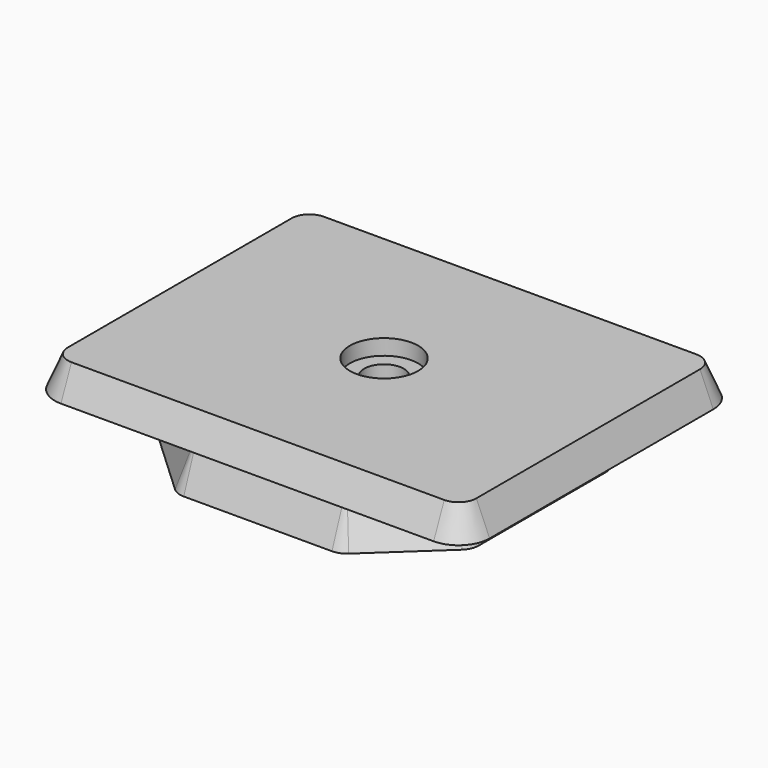
from build123d import *

# Parameters (mm, degrees)
F1_DEPTH       = 8.15
F1_TAPER       = 20
F2_T           = -4
F4_DEPTH       = 5
F4_TAPER       = 23
F6_D           = 6.35
F6_CBORE_D     = 11
F6_CBORE_DEPTH = 2.5


with BuildPart() as f1:
    # F0 (on Top) → F1 (new body)
    with BuildSketch(Plane.XY):
        with BuildLine():
            ThreePointArc((13.5235004185, 24.6379186874), (12.605417789, 25.1846935831), (11.5539321881, 25.375))
            Line((11.5539321881, 25.375), (-12.9567069347, 25.375))
            ThreePointArc((-12.9567069347, 25.375), (-14.1999477217, 25.1052659844), (-15.2196256222, 24.3445682304))
            Line((-15.2196256222, 24.3445682304), (-24.6379186874, 13.5235004185))
            ThreePointArc((-24.6379186874, 13.5235004185), (-25.1846935831, 12.605417789), (-25.375, 11.5539321881))
            Line((-25.375, 11.5539321881), (-25.375, -12.6529412227))
            ThreePointArc((-25.375, -12.6529412227), (-25.1255957189, -13.8505318001), (-24.4188512059, -14.8489995662))
            Line((-24.4188512059, -14.8489995662), (-13.972783394, -24.5710583435))
            ThreePointArc((-13.972783394, -24.5710583435), (-13.0270726549, -25.1667893035), (-11.9289321881, -25.375))
            Line((-11.9289321881, -25.375), (11.9289321881, -25.375))
            ThreePointArc((11.9289321881, -25.375), (13.0270726549, -25.1667893035), (13.972783394, -24.5710583435))
            Line((13.972783394, -24.5710583435), (24.4188512059, -14.8489995662))
            ThreePointArc((24.4188512059, -14.8489995662), (25.1255957189, -13.8505318001), (25.375, -12.6529412227))
            Line((25.375, -12.6529412227), (25.375, 12.9567069347))
            ThreePointArc((25.375, 12.9567069347), (25.1052659844, 14.1999477217), (24.3445682304, 15.2196256222))
            Line((24.3445682304, 15.2196256222), (13.5235004185, 24.6379186874))
        make_face()
    extrude(amount=F1_DEPTH, taper=F1_TAPER)

    # F2
    f2_openings = [f1.faces().sort_by_distance(p)[0] for p in [
        (0.016382, 0.006023, 0),
    ]]
    offset(amount=F2_T, openings=f2_openings)

    # F3 (on face) → F4 (join)
    with BuildSketch(Plane.XY.offset(8.15)):
        with BuildLine():
            ThreePointArc((35, 22.5), (33.5355339059, 26.0355339059), (30, 27.5))
            Line((30, 27.5), (-30, 27.5))
            ThreePointArc((-30, 27.5), (-33.5355339059, 26.0355339059), (-35, 22.5))
            Line((-35, 22.5), (-35, -22.5))
            ThreePointArc((-35, -22.5), (-33.5355339059, -26.0355339059), (-30, -27.5))
            Line((-30, -27.5), (30, -27.5))
            ThreePointArc((30, -27.5), (33.5355339059, -26.0355339059), (35, -22.5))
            Line((35, -22.5), (35, 22.5))
        make_face()
        with BuildLine():
            Line((11.5760193141, 22.4003768158), (22.397087126, 12.9820837505))
            ThreePointArc((22.397087126, 12.9820837505), (22.4056177404, 12.9706488817), (22.4086425907, 12.9567069347))
            Line((22.4086425907, 12.9567069347), (22.4086425907, -12.6529412227))
            ThreePointArc((22.4086425907, -12.6529412227), (22.405845722, -12.6663712392), (22.3979201499, -12.6775682533))
            Line((22.3979201499, -12.6775682533), (11.951852338, -22.3996270307))
            ThreePointArc((11.951852338, -22.3996270307), (11.9412469516, -22.406307675), (11.9289321881, -22.4086425907))
            Line((11.9289321881, -22.4086425907), (-11.9289321881, -22.4086425907))
            ThreePointArc((-11.9289321881, -22.4086425907), (-11.9412469516, -22.406307675), (-11.951852338, -22.3996270307))
            Line((-11.951852338, -22.3996270307), (-22.3979201499, -12.6775682533))
            ThreePointArc((-22.3979201499, -12.6775682533), (-22.405845722, -12.6663712392), (-22.4086425907, -12.6529412227))
            Line((-22.4086425907, -12.6529412227), (-22.4086425907, 11.5539321881))
            ThreePointArc((-22.4086425907, 11.5539321881), (-22.4065084571, 11.5657237547), (-22.4003768158, 11.5760193141))
            Line((-22.4003768158, 11.5760193141), (-12.9820837505, 22.397087126))
            ThreePointArc((-12.9820837505, 22.397087126), (-12.9706488817, 22.4056177404), (-12.9567069347, 22.4086425907))
            Line((-12.9567069347, 22.4086425907), (11.5539321881, 22.4086425907))
            ThreePointArc((11.5539321881, 22.4086425907), (11.5657237547, 22.4065084571), (11.5760193141, 22.4003768158))
        make_face(mode=Mode.SUBTRACT)
        with BuildLine():
            ThreePointArc((22.4086425907, 12.9567069347), (22.4056177404, 12.9706488817), (22.397087126, 12.9820837505))
            Line((22.397087126, 12.9820837505), (11.5760193141, 22.4003768158))
            ThreePointArc((11.5760193141, 22.4003768158), (11.5657237547, 22.4065084571), (11.5539321881, 22.4086425907))
            Line((11.5539321881, 22.4086425907), (-12.9567069347, 22.4086425907))
            ThreePointArc((-12.9567069347, 22.4086425907), (-12.9706488817, 22.4056177404), (-12.9820837505, 22.397087126))
            Line((-12.9820837505, 22.397087126), (-22.4003768158, 11.5760193141))
            ThreePointArc((-22.4003768158, 11.5760193141), (-22.4065084571, 11.5657237547), (-22.4086425907, 11.5539321881))
            Line((-22.4086425907, 11.5539321881), (-22.4086425907, -12.6529412227))
            ThreePointArc((-22.4086425907, -12.6529412227), (-22.405845722, -12.6663712392), (-22.3979201499, -12.6775682533))
            Line((-22.3979201499, -12.6775682533), (-11.951852338, -22.3996270307))
            ThreePointArc((-11.951852338, -22.3996270307), (-11.9412469516, -22.406307675), (-11.9289321881, -22.4086425907))
            Line((-11.9289321881, -22.4086425907), (11.9289321881, -22.4086425907))
            ThreePointArc((11.9289321881, -22.4086425907), (11.9412469516, -22.406307675), (11.951852338, -22.3996270307))
            Line((11.951852338, -22.3996270307), (22.3979201499, -12.6775682533))
            ThreePointArc((22.3979201499, -12.6775682533), (22.405845722, -12.6663712392), (22.4086425907, -12.6529412227))
            Line((22.4086425907, -12.6529412227), (22.4086425907, 12.9567069347))
        make_face()
    extrude(amount=F4_DEPTH, taper=F4_TAPER)

    # F6 (through all)
    with Locations(Plane.XY.offset(13.15)):
        with Locations((0, 0)):
            CounterBoreHole(F6_D / 2, F6_CBORE_D / 2, F6_CBORE_DEPTH)


solid = f1.part
